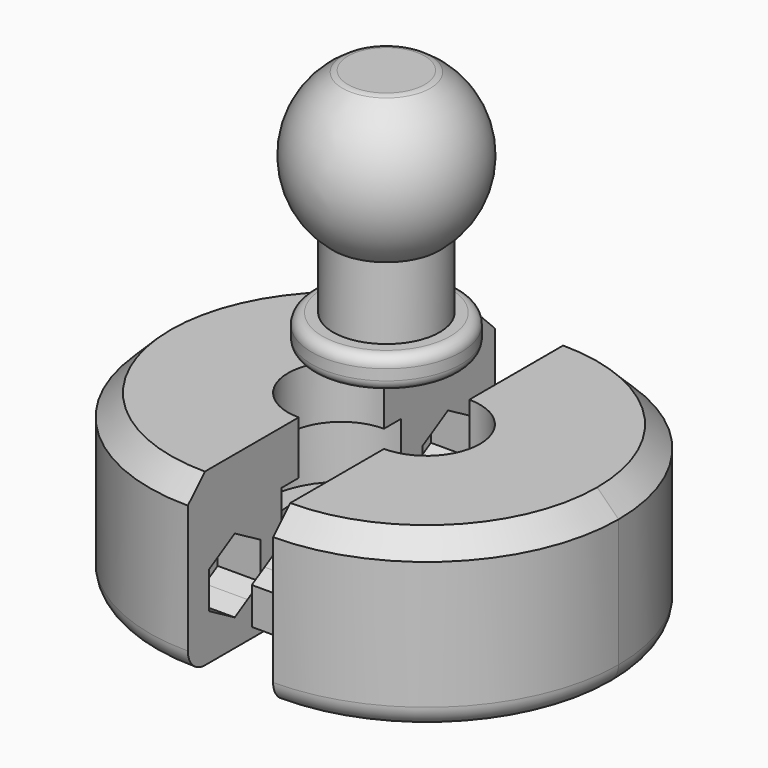
from build123d import *

# Parameters (mm, degrees)
F0_W           = 18
F0_H           = 8
F1_DEPTH       = 9
F3_DEPTH       = 4
F4_DEPTH       = 2.5
F6_R           = 8.99999
F8_DEPTH       = 2
F10_DEPTH      = 4
F11_DEPTH      = 2.5
F15_R          = 0.5
F17_DEPTH      = 4
F18_T1_DEPTH   = 2.50001
F18_T3_DEPTH   = 2e-05
F18_T6_ANGLE   = 90
F18_T8_ANGLE   = 90
F18_2_T1_DEPTH = 2.50001
F18_2_T3_DEPTH = 2e-05
F18_2_T6_ANGLE = 90
F18_2_T8_ANGLE = 90
F19_T1_DEPTH   = 2.571692988
F19_T3_DEPTH   = 2e-05
F19_T6_ANGLE   = 90
F19_T8_ANGLE   = 90
F19_2_T1_DEPTH = 2.571692988
F19_2_T3_DEPTH = 2e-05
F19_2_T6_ANGLE = 90
F19_2_T8_ANGLE = 90


# Not quite as in the source:
# - a fillet or chamfer that OpenCascade refuses, or shapes differently, is made with other operations: its cross-section is extruded or revolved along the edge and cut away or added
# - a fillet or chamfer is up to 0.001 mm smaller than in the source, because OpenCascade refuses the exact size


with BuildPart() as f1:
    # F0 (on Right) → F1 (new body)
    with BuildSketch(Plane.YZ):
        with Locations((-9, 4)):
            Rectangle(F0_W, F0_H)
    extrude(amount=F1_DEPTH)

    # F2 (on face) → F3 (cut)
    with BuildSketch(Plane(origin=(0, 0, 0), x_dir=(1, 0, 0), z_dir=(0, 0, -1))):
        with BuildLine():
            Line((9, 6.5), (9, 11.5))
            ThreePointArc((9, 11.5), (6.5, 9), (9, 6.5))
        make_face()
        with BuildLine():
            ThreePointArc((9, 6.5), (6.5, 9), (9, 11.5))
            Line((9, 11.5), (9, 12.5))
            ThreePointArc((9, 12.5), (5.5, 9), (9, 5.5))
            Line((9, 5.5), (9, 6.5))
        make_face()
    extrude(amount=-F3_DEPTH, mode=Mode.SUBTRACT)

    # F2 (on face) → F4 (join)
    with BuildSketch(Plane(origin=(0, 0, 0), x_dir=(1, 0, 0), z_dir=(0, 0, -1))):
        with BuildLine():
            ThreePointArc((9, 6.5), (6.5, 9), (9, 11.5))
            Line((9, 11.5), (9, 12.5))
            ThreePointArc((9, 12.5), (5.5, 9), (9, 5.5))
            Line((9, 5.5), (9, 6.5))
        make_face()
    extrude(amount=-F4_DEPTH)

    # F6 (radius 9 in the source; OpenCascade refuses exactly that, so slightly less here)
    f6_edges = [f1.edges().sort_by_distance(p)[0] for p in [
        (0, -18, 4),
        (0, 0, 4),
    ]]
    fillet(f6_edges, radius=F6_R)

    # F7 (on face) → F8 (cut)
    with BuildSketch(Plane.YZ.offset(9)):
        with BuildLine():
            ThreePointArc((-14.5000000001, 1.7009618943), (-13.9509618944, 2.2499999999), (-13.75, 3))
            ThreePointArc((-13.75, 3), (-13.9509618878, 3.7499999887), (-14.4999999775, 4.2990380927))
            ThreePointArc((-14.4999999775, 4.2990380927), (-15.2499999828, 4.5), (-15.9999999928, 4.2990381098))
            ThreePointArc((-15.9999999928, 4.2990381098), (-16.5490381036, 3.7500000036), (-16.75, 3))
            ThreePointArc((-16.75, 3), (-16.5490381076, 2.2500000033), (-16.0000000065, 1.7009618981))
            ThreePointArc((-16.0000000065, 1.7009618981), (-15.2500000038, 1.5), (-14.5000000001, 1.7009618943))
        make_face()
        with BuildLine():
            Line((-13.75, 2.1339745962), (-13.75, 3))
            ThreePointArc((-13.75, 3), (-13.9509618944, 2.2499999999), (-14.5000000001, 1.7009618943))
            Line((-14.5000000001, 1.7009618943), (-13.75, 2.1339745962))
        make_face()
        with BuildLine():
            ThreePointArc((-14.4999999775, 4.2990380927), (-13.9509618878, 3.7499999887), (-13.75, 3))
            Line((-13.75, 3), (-13.75, 3.8660254038))
            Line((-13.75, 3.8660254038), (-14.4999999775, 4.2990380927))
        make_face()
        with BuildLine():
            ThreePointArc((-15.9999999928, 4.2990381098), (-15.2499999828, 4.5), (-14.4999999775, 4.2990380927))
            Line((-14.4999999775, 4.2990380927), (-15.25, 4.7320508076))
            Line((-15.25, 4.7320508076), (-15.9999999928, 4.2990381098))
        make_face()
        with BuildLine():
            Line((-15.25, 1.2679491924), (-14.5000000001, 1.7009618943))
            ThreePointArc((-14.5000000001, 1.7009618943), (-15.2500000038, 1.5), (-16.0000000065, 1.7009618981))
            Line((-16.0000000065, 1.7009618981), (-15.25, 1.2679491924))
        make_face()
        with BuildLine():
            ThreePointArc((-16.75, 3), (-16.5490381036, 3.7500000036), (-15.9999999928, 4.2990381098))
            Line((-15.9999999928, 4.2990381098), (-16.75, 3.8660254038))
            Line((-16.75, 3.8660254038), (-16.75, 3))
        make_face()
        with BuildLine():
            Line((-16.75, 2.1339745962), (-16.0000000065, 1.7009618981))
            ThreePointArc((-16.0000000065, 1.7009618981), (-16.5490381076, 2.2500000033), (-16.75, 3))
            Line((-16.75, 3), (-16.75, 2.1339745962))
        make_face()
        with BuildLine():
            Line((-3.5000000108, 1.7009619005), (-2.75, 1.2679491924))
            Line((-2.75, 1.2679491924), (-1.9999999902, 1.7009619))
            ThreePointArc((-1.9999999902, 1.7009619), (-2.7500000006, 1.5), (-3.5000000108, 1.7009619005))
        make_face()
        with BuildLine():
            ThreePointArc((-1.25, 3), (-1.4509618915, 2.2500000049), (-1.9999999902, 1.7009619))
            Line((-1.9999999902, 1.7009619), (-1.25, 2.1339745962))
            Line((-1.25, 2.1339745962), (-1.25, 3))
        make_face()
        with BuildLine():
            ThreePointArc((-3.5000000108, 1.7009619005), (-2.7500000006, 1.5), (-1.9999999902, 1.7009619))
            ThreePointArc((-1.9999999902, 1.7009619), (-1.4509618915, 2.2500000049), (-1.25, 3))
            ThreePointArc((-1.25, 3), (-1.4509618964, 3.7500000036), (-2.0000000072, 4.2990381098))
            ThreePointArc((-2.0000000072, 4.2990381098), (-2.749999993, 4.5), (-3.4999999807, 4.2990381168))
            ThreePointArc((-3.4999999807, 4.2990381168), (-4.0490381001, 3.7500000097), (-4.25, 3))
            ThreePointArc((-4.25, 3), (-4.0490381088, 2.2500000054), (-3.5000000108, 1.7009619005))
        make_face()
        with BuildLine():
            Line((-4.25, 2.1339745962), (-3.5000000108, 1.7009619005))
            ThreePointArc((-3.5000000108, 1.7009619005), (-4.0490381088, 2.2500000054), (-4.25, 3))
            Line((-4.25, 3), (-4.25, 2.1339745962))
        make_face()
        with BuildLine():
            ThreePointArc((-2.0000000072, 4.2990381098), (-1.4509618964, 3.7500000036), (-1.25, 3))
            Line((-1.25, 3), (-1.25, 3.8660254038))
            Line((-1.25, 3.8660254038), (-2.0000000072, 4.2990381098))
        make_face()
        with BuildLine():
            Line((-4.25, 3.8660254038), (-4.25, 3))
            ThreePointArc((-4.25, 3), (-4.0490381001, 3.7500000097), (-3.4999999807, 4.2990381168))
            Line((-3.4999999807, 4.2990381168), (-4.25, 3.8660254038))
        make_face()
        with BuildLine():
            ThreePointArc((-3.4999999807, 4.2990381168), (-2.749999993, 4.5), (-2.0000000072, 4.2990381098))
            Line((-2.0000000072, 4.2990381098), (-2.75, 4.7320508076))
            Line((-2.75, 4.7320508076), (-3.4999999807, 4.2990381168))
        make_face()
    extrude(amount=-F8_DEPTH, mode=Mode.SUBTRACT)

    # F9 (on face) → F10 (cut)
    with BuildSketch(Plane.XY.offset(8)):
        with BuildLine():
            Line((9, -11.5), (9, -6.5))
            ThreePointArc((9, -6.5), (6.5, -9), (9, -11.5))
        make_face()
        with BuildLine():
            ThreePointArc((9, -11.5), (6.5, -9), (9, -6.5))
            Line((9, -6.5), (9, -5.5))
            ThreePointArc((9, -5.5), (5.5, -9), (9, -12.5))
            Line((9, -12.5), (9, -11.5))
        make_face()
    extrude(amount=-F10_DEPTH, mode=Mode.SUBTRACT)

    # F9 (on face) → F11 (join)
    with BuildSketch(Plane.XY.offset(8)):
        with BuildLine():
            ThreePointArc((9, -11.5), (6.5, -9), (9, -6.5))
            Line((9, -6.5), (9, -5.5))
            ThreePointArc((9, -5.5), (5.5, -9), (9, -12.5))
            Line((9, -12.5), (9, -11.5))
        make_face()
    extrude(amount=-F11_DEPTH)


with BuildPart() as f14:
    # F13 (on offset) → F14 (revolve)
    with BuildSketch(Plane.YZ.offset(11)):
        with BuildLine():
            Line((-12.3604685068, 10.4050319642), (-8.8604685068, 10.4050319642))
            Line((-8.8604685068, 10.4050319642), (-8.8604685068, 21.9050319642))
            Line((-8.8604685068, 21.9050319642), (-10.7969601799, 21.9050319642))
            ThreePointArc((-10.7969601799, 21.9050319642), (-12.846066058, 18.7441663918), (-11.3604685068, 15.282532965))
            Line((-11.3604685068, 15.282532965), (-11.3604685068, 14.4050319642))
            Line((-11.3604685068, 14.4050319642), (-11.3604685068, 11.9050319642))
            Line((-11.3604685068, 11.9050319642), (-12.3604685068, 11.9050319642))
            Line((-12.3604685068, 11.9050319642), (-12.3604685068, 10.4050319642))
        make_face()
    revolve(axis=Axis((11, -8.8604685068, 16.1550319642), (0, 0, -1)))

    # F15
    f15_edges = [f14.edges().sort_by_distance(p)[0] for p in [
        (11, -5.360469, 11.905032),
        (11, -5.360469, 10.405032),
        (11, -12.360469, 11.155032),
        (11, -6.923977, 21.905032),
    ]]
    fillet(f15_edges, radius=F15_R)


with BuildPart() as f16_1:
    # F16: instance of F1
    add(f1.part.mirror(Plane.YZ.offset(11)))

    # F17 (add): faces of the model
    f17_faces = [f16_1.faces().sort_by_distance(p)[0] for p in [
        (15, -15.25, 3),
        (15, -2.75, 3),
    ]]
    extrude(f17_faces, amount=F17_DEPTH)

    # F18#2: fillet of radius 1 on 1 edges, made by hand

    # F18_2_s2 → F18_2_t1 (cut)
    with BuildSketch(Plane.YZ.offset(10.5)):
        with BuildLine():
            ThreePointArc((-1, 0), (-0.2928932188, 0.2928932188), (0, 1))
            Line((0, 1), (0, 0))
            Line((0, 0), (-1, 0))
        make_face()
        with BuildLine():
            ThreePointArc((-17, 0), (-17.7071067812, 0.2928932188), (-18, 1))
            Line((-18, 1), (-18, 0))
            Line((-18, 0), (-17, 0))
        make_face()
    extrude(amount=F18_2_T1_DEPTH, mode=Mode.SUBTRACT)

    # F18_2_s4 → F18_2_t3 (cut)
    with BuildSketch(Plane.XZ.offset(8.99999)):
        with BuildLine():
            ThreePointArc((21, 0), (21.7071067812, 0.2928932188), (22, 1))
            Line((22, 1), (22, 0))
            Line((22, 0), (21, 0))
        make_face()
    extrude(amount=F18_2_T3_DEPTH, mode=Mode.SUBTRACT)

    # F18_2_s5 → F18_2_t6 (revolve, cut)
    with BuildSketch(Plane.YZ.offset(13.00001)):
        with BuildLine():
            ThreePointArc((-1, 0), (-0.2928932188, 0.2928932188), (0, 1))
            Line((0, 1), (0, 0))
            Line((0, 0), (-1, 0))
        make_face()
    revolve(axis=Axis((13.00001, -8.99999, 0), (0, 0, -1)), revolution_arc=F18_2_T6_ANGLE, mode=Mode.SUBTRACT)

    # F18_2_s7 → F18_2_t8 (revolve, cut)
    with BuildSketch(Plane.YZ.offset(13.00001)):
        with BuildLine():
            ThreePointArc((-17, 0), (-17.7071067812, 0.2928932188), (-18, 1))
            Line((-18, 1), (-18, 0))
            Line((-18, 0), (-17, 0))
        make_face()
    revolve(axis=Axis((13.00001, -9.00001, 0), (0, 0, 1)), revolution_arc=F18_2_T8_ANGLE, mode=Mode.SUBTRACT)

    # F19#2: chamfer of 1 on 1 edges, made by hand

    # F19_2_s2 → F19_2_t1 (cut)
    with BuildSketch(Plane.YZ.offset(10.428317012)):
        Polygon((0, 7), (-1, 8), (0, 8), align=None)
        Polygon((-17, 8), (-18, 7), (-18, 8), align=None)
    extrude(amount=F19_2_T1_DEPTH, mode=Mode.SUBTRACT)

    # F19_2_s4 → F19_2_t3 (cut)
    with BuildSketch(Plane.XZ.offset(8.99999)):
        Polygon((22, 7), (21, 8), (22, 8), align=None)
    extrude(amount=F19_2_T3_DEPTH, mode=Mode.SUBTRACT)

    # F19_2_s5 → F19_2_t6 (revolve, cut)
    with BuildSketch(Plane.YZ.offset(13.00001)):
        Polygon((0, 7), (-1, 8), (0, 8), align=None)
    revolve(axis=Axis((13.00001, -8.99999, 8), (0, 0, -1)), revolution_arc=F19_2_T6_ANGLE, mode=Mode.SUBTRACT)

    # F19_2_s7 → F19_2_t8 (revolve, cut)
    with BuildSketch(Plane.YZ.offset(13.00001)):
        Polygon((-17, 8), (-18, 7), (-18, 8), align=None)
    revolve(axis=Axis((13.00001, -9.00001, 8), (0, 0, 1)), revolution_arc=F19_2_T8_ANGLE, mode=Mode.SUBTRACT)


with BuildPart() as f1_1:
    add(f1.part)

    # F18: fillet of radius 1 on 1 edges, made by hand

    # F18_s2 → F18_t1 (cut)
    with BuildSketch(Plane.YZ.offset(8.99999)):
        with BuildLine():
            ThreePointArc((-1, 0), (-0.2928932188, 0.2928932188), (0, 1))
            Line((0, 1), (0, 0))
            Line((0, 0), (-1, 0))
        make_face()
        with BuildLine():
            ThreePointArc((-17, 0), (-17.7071067812, 0.2928932188), (-18, 1))
            Line((-18, 1), (-18, 0))
            Line((-18, 0), (-17, 0))
        make_face()
    extrude(amount=F18_T1_DEPTH, mode=Mode.SUBTRACT)

    # F18_s4 → F18_t3 (cut)
    with BuildSketch(Plane.XZ.offset(8.99999)):
        with BuildLine():
            ThreePointArc((1, 0), (0.2928932188, 0.2928932188), (0, 1))
            Line((0, 1), (0, 0))
            Line((0, 0), (1, 0))
        make_face()
    extrude(amount=F18_T3_DEPTH, mode=Mode.SUBTRACT)

    # F18_s5 → F18_t6 (revolve, cut)
    with BuildSketch(Plane.YZ.offset(8.99999)):
        with BuildLine():
            ThreePointArc((-1, 0), (-0.2928932188, 0.2928932188), (0, 1))
            Line((0, 1), (0, 0))
            Line((0, 0), (-1, 0))
        make_face()
    revolve(axis=Axis((8.99999, -8.99999, 0), (0, 0, 1)), revolution_arc=F18_T6_ANGLE, mode=Mode.SUBTRACT)

    # F18_s7 → F18_t8 (revolve, cut)
    with BuildSketch(Plane.YZ.offset(8.99999)):
        with BuildLine():
            ThreePointArc((-17, 0), (-17.7071067812, 0.2928932188), (-18, 1))
            Line((-18, 1), (-18, 0))
            Line((-18, 0), (-17, 0))
        make_face()
    revolve(axis=Axis((8.99999, -9.00001, 0), (0, 0, -1)), revolution_arc=F18_T8_ANGLE, mode=Mode.SUBTRACT)

    # F19: chamfer of 1 on 1 edges, made by hand

    # F19_s2 → F19_t1 (cut)
    with BuildSketch(Plane.YZ.offset(8.99999)):
        Polygon((0, 7), (-1, 8), (0, 8), align=None)
        Polygon((-17, 8), (-18, 7), (-18, 8), align=None)
    extrude(amount=F19_T1_DEPTH, mode=Mode.SUBTRACT)

    # F19_s4 → F19_t3 (cut)
    with BuildSketch(Plane.XZ.offset(8.99999)):
        Polygon((0, 7), (1, 8), (0, 8), align=None)
    extrude(amount=F19_T3_DEPTH, mode=Mode.SUBTRACT)

    # F19_s5 → F19_t6 (revolve, cut)
    with BuildSketch(Plane.YZ.offset(8.99999)):
        Polygon((0, 7), (-1, 8), (0, 8), align=None)
    revolve(axis=Axis((8.99999, -8.99999, 8), (0, 0, 1)), revolution_arc=F19_T6_ANGLE, mode=Mode.SUBTRACT)

    # F19_s7 → F19_t8 (revolve, cut)
    with BuildSketch(Plane.YZ.offset(8.99999)):
        Polygon((-17, 8), (-18, 7), (-18, 8), align=None)
    revolve(axis=Axis((8.99999, -9.00001, 8), (0, 0, -1)), revolution_arc=F19_T8_ANGLE, mode=Mode.SUBTRACT)


solid = Compound([f14.part, f16_1.part, f1_1.part])
